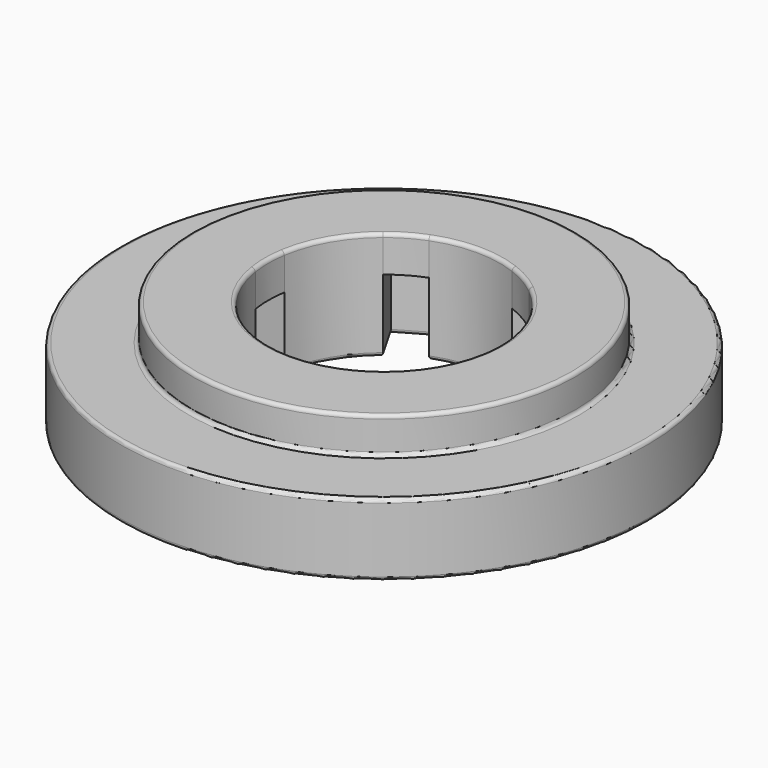
from build123d import *

# Parameters (mm, degrees)
F0_R     = 36.5
F0_R_2   = 26.5
F1_DEPTH = 10
F2_DEPTH = 15
F3_DEPTH = 10
F4_R     = 0.5


with BuildPart() as f1:
    # F0 (on Top) → F1 (new body)
    with BuildSketch(Plane.XY):
        Circle(F0_R)
        Circle(F0_R_2, mode=Mode.SUBTRACT)
        Circle(F0_R_2)
        with BuildLine():
            ThreePointArc((10.066804, 12.436216), (13.856406, 8), (15.803481, 2.5))
            Line((15.803481, 2.5), (21.303481, 2.5))
            Line((21.303481, 2.5), (21.303481, -2.5))
            Line((21.303481, -2.5), (15.803481, -2.5))
            ThreePointArc((15.803481, -2.5), (13.856406, -8), (10.066804, -12.436216))
            Line((10.066804, -12.436216), (12.816804, -17.199355))
            Line((12.816804, -17.199355), (8.486677, -19.699355))
            Line((8.486677, -19.699355), (5.736677, -14.936216))
            ThreePointArc((5.736677, -14.936216), (0, -16), (-5.736677, -14.936216))
            Line((-5.736677, -14.936216), (-8.486677, -19.699355))
            Line((-8.486677, -19.699355), (-12.816804, -17.199355))
            Line((-12.816804, -17.199355), (-10.066804, -12.436216))
            ThreePointArc((-10.066804, -12.436216), (-13.856406, -8), (-15.803481, -2.5))
            Line((-15.803481, -2.5), (-21.303481, -2.5))
            Line((-21.303481, -2.5), (-21.303481, 2.5))
            Line((-21.303481, 2.5), (-15.803481, 2.5))
            ThreePointArc((-15.803481, 2.5), (-13.856406, 8), (-10.066804, 12.436216))
            Line((-10.066804, 12.436216), (-12.816804, 17.199355))
            Line((-12.816804, 17.199355), (-8.486677, 19.699355))
            Line((-8.486677, 19.699355), (-5.736677, 14.936216))
            ThreePointArc((-5.736677, 14.936216), (0, 16), (5.736677, 14.936216))
            Line((5.736677, 14.936216), (8.486677, 19.699355))
            Line((8.486677, 19.699355), (12.816804, 17.199355))
            Line((12.816804, 17.199355), (10.066804, 12.436216))
        make_face(mode=Mode.SUBTRACT)
        with BuildLine():
            ThreePointArc((-10.066804, 12.436216), (-8, 13.856406), (-5.736677, 14.936216))
            Line((-5.736677, 14.936216), (-8.486677, 19.699355))
            Line((-8.486677, 19.699355), (-12.816804, 17.199355))
            Line((-12.816804, 17.199355), (-10.066804, 12.436216))
        make_face()
        with BuildLine():
            ThreePointArc((5.736677, 14.936216), (8, 13.856406), (10.066804, 12.436216))
            Line((10.066804, 12.436216), (12.816804, 17.199355))
            Line((12.816804, 17.199355), (8.486677, 19.699355))
            Line((8.486677, 19.699355), (5.736677, 14.936216))
        make_face()
        with BuildLine():
            ThreePointArc((15.803481, 2.5), (15.950794, 1.253856), (16, 0))
            ThreePointArc((16, 0), (15.950794, -1.253856), (15.803481, -2.5))
            Line((15.803481, -2.5), (21.303481, -2.5))
            Line((21.303481, -2.5), (21.303481, 2.5))
            Line((21.303481, 2.5), (15.803481, 2.5))
        make_face()
        with BuildLine():
            Line((12.816804, -17.199355), (10.066804, -12.436216))
            ThreePointArc((10.066804, -12.436216), (8, -13.856406), (5.736677, -14.936216))
            Line((5.736677, -14.936216), (8.486677, -19.699355))
            Line((8.486677, -19.699355), (12.816804, -17.199355))
        make_face()
        with BuildLine():
            Line((-8.486677, -19.699355), (-5.736677, -14.936216))
            ThreePointArc((-5.736677, -14.936216), (-8, -13.856406), (-10.066804, -12.436216))
            Line((-10.066804, -12.436216), (-12.816804, -17.199355))
            Line((-12.816804, -17.199355), (-8.486677, -19.699355))
        make_face()
        with BuildLine():
            ThreePointArc((-15.803481, -2.5), (-16, 0), (-15.803481, 2.5))
            Line((-15.803481, 2.5), (-21.303481, 2.5))
            Line((-21.303481, 2.5), (-21.303481, -2.5))
            Line((-21.303481, -2.5), (-15.803481, -2.5))
        make_face()
    extrude(amount=F1_DEPTH)

    # F0 (on Top) → F2 (join)
    with BuildSketch(Plane.XY):
        Circle(F0_R_2)
        with BuildLine():
            ThreePointArc((10.066804, 12.436216), (13.856406, 8), (15.803481, 2.5))
            Line((15.803481, 2.5), (21.303481, 2.5))
            Line((21.303481, 2.5), (21.303481, -2.5))
            Line((21.303481, -2.5), (15.803481, -2.5))
            ThreePointArc((15.803481, -2.5), (13.856406, -8), (10.066804, -12.436216))
            Line((10.066804, -12.436216), (12.816804, -17.199355))
            Line((12.816804, -17.199355), (8.486677, -19.699355))
            Line((8.486677, -19.699355), (5.736677, -14.936216))
            ThreePointArc((5.736677, -14.936216), (0, -16), (-5.736677, -14.936216))
            Line((-5.736677, -14.936216), (-8.486677, -19.699355))
            Line((-8.486677, -19.699355), (-12.816804, -17.199355))
            Line((-12.816804, -17.199355), (-10.066804, -12.436216))
            ThreePointArc((-10.066804, -12.436216), (-13.856406, -8), (-15.803481, -2.5))
            Line((-15.803481, -2.5), (-21.303481, -2.5))
            Line((-21.303481, -2.5), (-21.303481, 2.5))
            Line((-21.303481, 2.5), (-15.803481, 2.5))
            ThreePointArc((-15.803481, 2.5), (-13.856406, 8), (-10.066804, 12.436216))
            Line((-10.066804, 12.436216), (-12.816804, 17.199355))
            Line((-12.816804, 17.199355), (-8.486677, 19.699355))
            Line((-8.486677, 19.699355), (-5.736677, 14.936216))
            ThreePointArc((-5.736677, 14.936216), (0, 16), (5.736677, 14.936216))
            Line((5.736677, 14.936216), (8.486677, 19.699355))
            Line((8.486677, 19.699355), (12.816804, 17.199355))
            Line((12.816804, 17.199355), (10.066804, 12.436216))
        make_face(mode=Mode.SUBTRACT)
        with BuildLine():
            ThreePointArc((-10.066804, 12.436216), (-8, 13.856406), (-5.736677, 14.936216))
            Line((-5.736677, 14.936216), (-8.486677, 19.699355))
            Line((-8.486677, 19.699355), (-12.816804, 17.199355))
            Line((-12.816804, 17.199355), (-10.066804, 12.436216))
        make_face()
        with BuildLine():
            ThreePointArc((5.736677, 14.936216), (8, 13.856406), (10.066804, 12.436216))
            Line((10.066804, 12.436216), (12.816804, 17.199355))
            Line((12.816804, 17.199355), (8.486677, 19.699355))
            Line((8.486677, 19.699355), (5.736677, 14.936216))
        make_face()
        with BuildLine():
            ThreePointArc((15.803481, 2.5), (15.950794, 1.253856), (16, 0))
            ThreePointArc((16, 0), (15.950794, -1.253856), (15.803481, -2.5))
            Line((15.803481, -2.5), (21.303481, -2.5))
            Line((21.303481, -2.5), (21.303481, 2.5))
            Line((21.303481, 2.5), (15.803481, 2.5))
        make_face()
        with BuildLine():
            Line((12.816804, -17.199355), (10.066804, -12.436216))
            ThreePointArc((10.066804, -12.436216), (8, -13.856406), (5.736677, -14.936216))
            Line((5.736677, -14.936216), (8.486677, -19.699355))
            Line((8.486677, -19.699355), (12.816804, -17.199355))
        make_face()
        with BuildLine():
            Line((-8.486677, -19.699355), (-5.736677, -14.936216))
            ThreePointArc((-5.736677, -14.936216), (-8, -13.856406), (-10.066804, -12.436216))
            Line((-10.066804, -12.436216), (-12.816804, -17.199355))
            Line((-12.816804, -17.199355), (-8.486677, -19.699355))
        make_face()
        with BuildLine():
            ThreePointArc((-15.803481, -2.5), (-16, 0), (-15.803481, 2.5))
            Line((-15.803481, 2.5), (-21.303481, 2.5))
            Line((-21.303481, 2.5), (-21.303481, -2.5))
            Line((-21.303481, -2.5), (-15.803481, -2.5))
        make_face()
    extrude(amount=F2_DEPTH)

    # F0 (on Top) → F3 (cut)
    with BuildSketch(Plane.XY):
        with BuildLine():
            ThreePointArc((5.736677, 14.936216), (8, 13.856406), (10.066804, 12.436216))
            Line((10.066804, 12.436216), (12.816804, 17.199355))
            Line((12.816804, 17.199355), (8.486677, 19.699355))
            Line((8.486677, 19.699355), (5.736677, 14.936216))
        make_face()
        with BuildLine():
            ThreePointArc((-10.066804, 12.436216), (-8, 13.856406), (-5.736677, 14.936216))
            Line((-5.736677, 14.936216), (-8.486677, 19.699355))
            Line((-8.486677, 19.699355), (-12.816804, 17.199355))
            Line((-12.816804, 17.199355), (-10.066804, 12.436216))
        make_face()
        with BuildLine():
            ThreePointArc((-15.803481, -2.5), (-16, 0), (-15.803481, 2.5))
            Line((-15.803481, 2.5), (-21.303481, 2.5))
            Line((-21.303481, 2.5), (-21.303481, -2.5))
            Line((-21.303481, -2.5), (-15.803481, -2.5))
        make_face()
        with BuildLine():
            Line((-8.486677, -19.699355), (-5.736677, -14.936216))
            ThreePointArc((-5.736677, -14.936216), (-8, -13.856406), (-10.066804, -12.436216))
            Line((-10.066804, -12.436216), (-12.816804, -17.199355))
            Line((-12.816804, -17.199355), (-8.486677, -19.699355))
        make_face()
        with BuildLine():
            Line((12.816804, -17.199355), (10.066804, -12.436216))
            ThreePointArc((10.066804, -12.436216), (8, -13.856406), (5.736677, -14.936216))
            Line((5.736677, -14.936216), (8.486677, -19.699355))
            Line((8.486677, -19.699355), (12.816804, -17.199355))
        make_face()
        with BuildLine():
            ThreePointArc((15.803481, 2.5), (15.950794, 1.253856), (16, 0))
            ThreePointArc((16, 0), (15.950794, -1.253856), (15.803481, -2.5))
            Line((15.803481, -2.5), (21.303481, -2.5))
            Line((21.303481, -2.5), (21.303481, 2.5))
            Line((21.303481, 2.5), (15.803481, 2.5))
        make_face()
    extrude(amount=F3_DEPTH, mode=Mode.SUBTRACT)

    # F4
    f4_edges = [f1.edges().sort_by_distance(p)[0] for p in [
        (-26.5, 0, 10),
        (-36.5, 0, 10),
        (-26.5, 0, 15),
        (15.803481, 2.5, 15),
        (-36.5, 0, 0),
        (13.856406, -8, 0),
        (0, -16, 0),
        (-13.856406, -8, 0),
        (-13.856406, 8, 0),
        (0, 16, 0),
        (13.856406, 8, 0),
        (-7.111677, -17.317786, 0),
        (-10.65174, -18.449355, 0),
        (-11.441804, -14.817786, 0),
        (-18.553481, -2.5, 0),
        (-21.303481, 0, 0),
        (-18.553481, 2.5, 0),
        (-11.441804, 14.817786, 0),
        (-10.65174, 18.449355, 0),
        (-7.111677, 17.317786, 0),
        (7.111677, 17.317786, 0),
        (10.65174, 18.449355, 0),
        (11.441804, 14.817786, 0),
        (18.553481, -2.5, 0),
        (21.303481, 0, 0),
        (18.553481, 2.5, 0),
        (11.441804, -14.817786, 0),
        (10.65174, -18.449355, 0),
        (7.111677, -17.317786, 0),
    ]]
    fillet(f4_edges, radius=F4_R)


solid = f1.part
